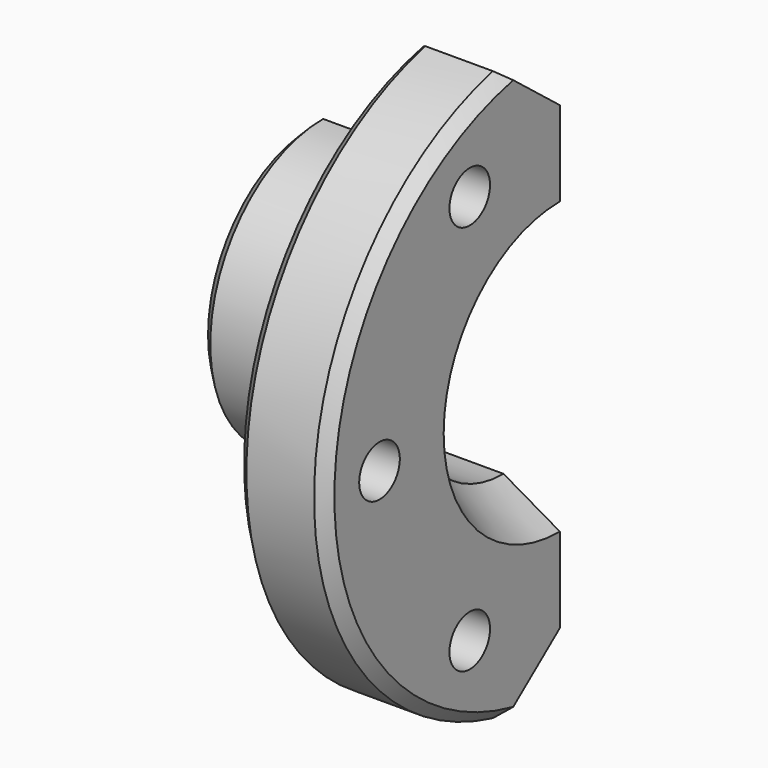
from build123d import *

# Parameters (mm, degrees)
F1_ANGLE    = 180
F2_R        = 4
F2_R_2      = 2.25
F3_DEPTH    = 4.5
F4_DEPTH    = 8
F5_SIZE     = 1
F6_T1_DEPTH = 37.8922901759


# Not quite as in the source:
# - a fillet or chamfer that OpenCascade refuses, or shapes differently, is made with other operations: its cross-section is extruded or revolved along the edge and cut away or added


with BuildPart() as f1:
    # F0 (on Front) → F1 (revolve)
    with BuildSketch(Plane.XZ):
        Polygon((0, 12.5), (0, 10), (17, 10), (22, 12.8867513459), (22, 26), (14, 26), (14, 12.5), align=None)
    revolve(axis=Axis((14.5569612949, 0, 0), (1, 0, 0)), revolution_arc=F1_ANGLE)

    # F2 (on face) → F3 (cut)
    with BuildSketch(Plane(origin=(14, 0, 0), x_dir=(0, -1, 0), z_dir=(-1, 0, 0))):
        with Locations((20, 0)):
            Circle(F2_R)
        with Locations((20, 0)):
            Circle(F2_R_2, mode=Mode.SUBTRACT)
        with Locations((10, -17.3205080757)):
            Circle(F2_R)
        with Locations((10, -17.3205080757)):
            Circle(F2_R_2, mode=Mode.SUBTRACT)
        with Locations((10, 17.3205080757)):
            Circle(F2_R)
        with Locations((10, 17.3205080757)):
            Circle(F2_R_2, mode=Mode.SUBTRACT)
    extrude(amount=-F3_DEPTH, mode=Mode.SUBTRACT)

    # F4 (cut): faces of the model
    f4_faces = [f1.faces().sort_by_distance(p)[0] for p in [
        (14, -10, 17.3205080757),
        (14, -20, 0),
        (14, -10, -17.3205080757),
    ]]
    extrude(f4_faces, amount=-F4_DEPTH, mode=Mode.SUBTRACT)

    # F5
    f5_edges = [f1.edges().sort_by_distance(p)[0] for p in [
        (0, -12.5, 0),
        (14, -26, 0),
        (22, -26, 0),
    ]]
    chamfer(f5_edges, length=F5_SIZE)

    # F6: chamfer of 5 on 2 edges, made by hand

    # F6_s2 → F6_t1 (cut)
    with BuildSketch(Plane.YZ.offset(-0.946145088)):
        with BuildLine():
            Line((0, -20.3960780544), (-6.1904761905, -25.2522871149))
            ThreePointArc((-6.1904761905, -25.2522871149), (-3.188239959, -25.8037812338), (0, -26))
            Line((0, -26), (0, -20.3960780544))
        make_face()
        with BuildLine():
            Line((0, 20.3960780544), (-6.1904761905, 25.2522871149))
            ThreePointArc((-6.1904761905, 25.2522871149), (-3.188239959, 25.8037812338), (0, 26))
            Line((0, 26), (0, 20.3960780544))
        make_face()
    extrude(amount=F6_T1_DEPTH, mode=Mode.SUBTRACT)


solid = f1.part
